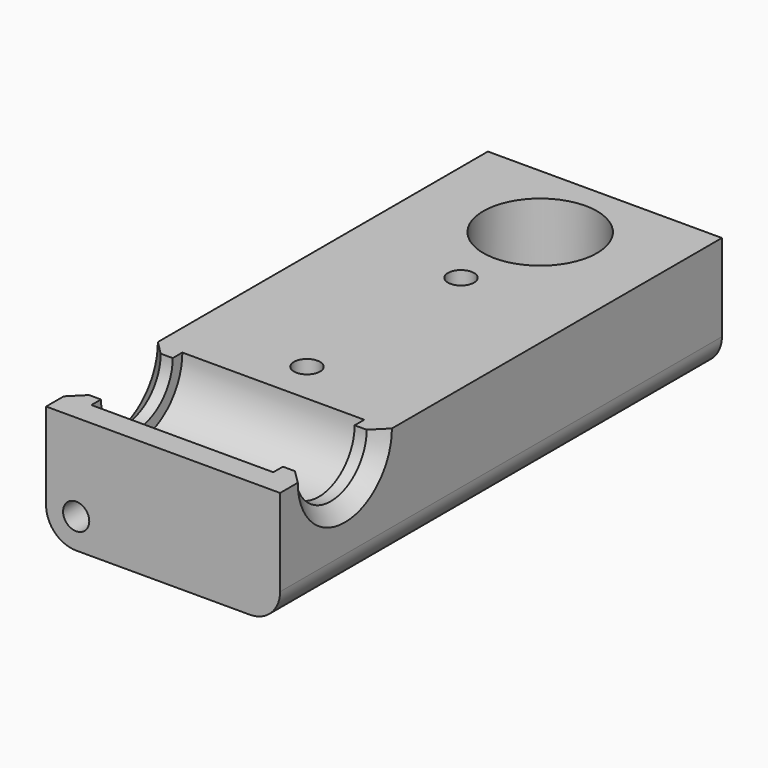
from build123d import *

# Parameters (mm, degrees)
F0_W      = 30.8750208
F0_H      = 72.8625058
F0_R      = 1.7272
F0_R_2    = 5.9124977
F1_DEPTH  = 3.437509
F2_W      = 30.8750208
F2_H      = 72.8625058
F2_R      = 1.7272
F2_R_2    = 7.5
F3_DEPTH  = 12
F4_W      = 24
F4_H      = 15
F5_DEPTH  = 7.5
F6_R      = 7.49999
F8_DEPTH  = 30.8750208
F9_R      = 3.96875
F10_DEPTH = 9.0875104
F11_R     = 3.96875
F12_R     = 1.7272
F13_DEPTH = 6.35
F14_SIZE  = 1.850009


# Not quite as in the source:
# - a fillet or chamfer is up to 0.001 mm smaller than in the source, because OpenCascade refuses the exact size


with BuildPart() as f1:
    # F0 (on Top) → F1 (new body)
    with BuildSketch(Plane.XY):
        with Locations((15.4375104, -36.4312529)):
            Rectangle(F0_W, F0_H)
        with Locations((15.4375104, -49.1312477)):
            Circle(F0_R, mode=Mode.SUBTRACT)
        with Locations((15.4375104, -23.7312477)):
            Circle(F0_R, mode=Mode.SUBTRACT)
        with Locations((15.4375104, -10.6749977)):
            Circle(F0_R_2, mode=Mode.SUBTRACT)
    extrude(amount=F1_DEPTH)

    # F2 (on face) → F3 (join)
    with BuildSketch(Plane.XY.offset(3.437509)):
        with Locations((15.4375104, -36.4312529)):
            Rectangle(F2_W, F2_H)
        with Locations((15.4375104, -49.1312477)):
            Circle(F2_R, mode=Mode.SUBTRACT)
        with Locations((15.4375104, -23.7312477)):
            Circle(F2_R, mode=Mode.SUBTRACT)
        with Locations((15.4375104, -10.6749977)):
            Circle(F2_R_2, mode=Mode.SUBTRACT)
    extrude(amount=F3_DEPTH)

    # F4 (on face) → F5 (cut)
    with BuildSketch(Plane.XY.offset(15.437509)):
        with Locations((15.4375104, -62.1875058)):
            Rectangle(F4_W, F4_H)
    extrude(amount=-F5_DEPTH, mode=Mode.SUBTRACT)

    # F6 (radius 7.5 in the source; OpenCascade refuses exactly that, so slightly less here)
    f6_edges = [f1.edges().sort_by_distance(p)[0] for p in [
        (15.43751, -54.687506, 7.937509),
        (15.43751, -69.687506, 7.937509),
    ]]
    fillet(f6_edges, radius=F6_R)

    # F7 (on face) → F8 (cut, through all)
    with BuildSketch(Plane(origin=(0, 0, 0), x_dir=(0, -1, 0), z_dir=(-1, 0, 0))):
        with BuildLine():
            Line((68.1000035, 15.437509), (56.2750081, 15.437509))
            ThreePointArc((56.2750081, 15.437509), (62.1875058, 9.5250113), (68.1000035, 15.437509))
        make_face()
    extrude(amount=-F8_DEPTH, mode=Mode.SUBTRACT)

    # F9 (on face) → F10 (cut)
    with BuildSketch(Plane(origin=(0, 0, 0), x_dir=(1, 0, 0), z_dir=(0, 0, -1))):
        with Locations((15.4375104, 23.7312477)):
            Circle(F9_R)
        with Locations((15.4375104, 49.1312477)):
            Circle(F9_R)
    extrude(amount=-F10_DEPTH, mode=Mode.SUBTRACT)

    # F11
    f11_edges = [f1.edges().sort_by_distance(p)[0] for p in [
        (0, -36.431253, 0),
        (30.875021, -36.431253, 0),
    ]]
    fillet(f11_edges, radius=F11_R)

    # F12 (on face) → F13 (cut)
    with BuildSketch(Plane.XZ.offset(72.8625058)):
        with Locations((3.96875, 3.96875)):
            Circle(F12_R)
    extrude(amount=-F13_DEPTH, mode=Mode.SUBTRACT)

    # F14
    f14_edges = [f1.edges().sort_by_distance(p)[0] for p in [
        (9.525013, -10.674998, 0),
        (30.875021, -62.187506, 9.525011),
        (0, -62.187506, 9.525011),
    ]]
    chamfer(f14_edges, length=F14_SIZE)


solid = f1.part
